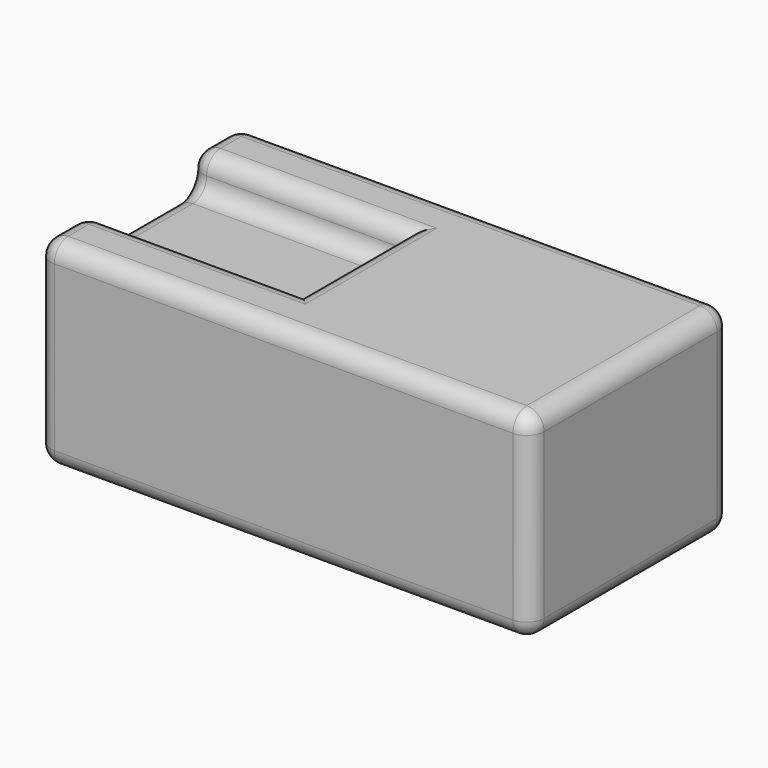
from build123d import *

# Parameters (mm, degrees)
F0_W     = 570
F0_H     = 290
F1_DEPTH = 230
F3_DEPTH = 40
F4_R     = 19.99999


# Not quite as in the source:
# - a fillet or chamfer is up to 0.001 mm smaller than in the source, because OpenCascade refuses the exact size
# - a feature of the source that left no trace in its solid (it failed there, or was rolled back) is left out


with BuildPart() as f1:
    # F0 (on Top) → F1 (new body)
    with BuildSketch(Plane.XY):
        with Locations((285, -145)):
            Rectangle(F0_W, F0_H)
    extrude(amount=F1_DEPTH)

    # F2 (on face) → F3 (cut)
    with BuildSketch(Plane.XY.offset(230)):
        Polygon((0, -220), (250, -220), (250, -145), (250, -70), (0, -70), (0, -145), align=None)
    extrude(amount=-F3_DEPTH, mode=Mode.SUBTRACT)

    # F4 (radius 20 in the source; OpenCascade refuses exactly that, so slightly less here)
    f4_edges = [f1.edges().sort_by_distance(p)[0] for p in [
        (0, -145, 0),
        (0, -290, 115),
        (0, -255, 230),
        (0, -220, 210),
        (0, -145, 190),
        (0, -70, 210),
        (0, -35, 230),
        (0, 0, 115),
        (570, -290, 115),
        (570, 0, 115),
        (570, -145, 0),
        (570, -145, 230),
        (285, -290, 0),
        (285, -290, 230),
        (285, 0, 0),
        (285, 0, 230),
        (125, -220, 190),
        (250, -145, 190),
        (125, -70, 190),
        (125, -220, 230),
        (250, -145, 230),
        (125, -70, 230),
    ]]
    fillet(f4_edges, radius=F4_R)


solid = f1.part
